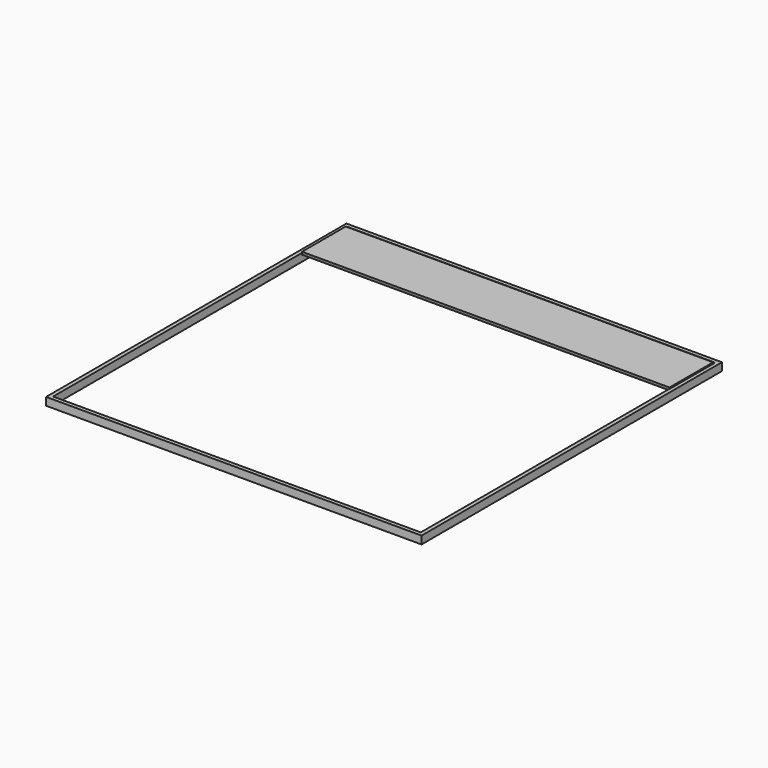
from build123d import *

# Parameters (mm, degrees)
F1_DEPTH  = 19.05
F2_W      = 895.35
F2_H      = 19.05
F5_DEPTH  = 19.05
F6_DEPTH  = 38.1
F3_W      = 895.35
F3_H      = 19.05
F7_DEPTH  = 19.05
F4_W      = 895.35
F4_H      = 19.05
F8_DEPTH  = 127
F10_W     = 895.35
F10_H     = 19.05
F11_DEPTH = 19.05
F12_W     = 895.35
F12_H     = 133.35
F13_DEPTH = 3.175
F13_TAPER = 3


# Not quite as in the source:
# - the program builds the solid bodies; features that only make, move or delete a surface that nothing else refers to are left out


with BuildPart() as f1:
    # F0 (on Top) → F1 (new body)
    with BuildSketch(Plane.XY):
        Polygon((457.2, -457.2), (457.2, 457.2), (186.2517595291, 457.2), (-457.2, 457.2), (-457.2, -457.2), align=None)
        Polygon((-447.675, 447.675), (186.2517595291, 447.675), (447.675, 447.675), (447.675, -447.675), (-447.675, -447.675), align=None, mode=Mode.SUBTRACT)
    extrude(amount=F1_DEPTH)

    # F3 (on face) → F7 (cut)
    with BuildSketch(Plane.XY.offset(19.05)):
        with Locations((0, 298.0556269322)):
            Rectangle(F3_W, F3_H)
    extrude(amount=-F7_DEPTH, mode=Mode.SUBTRACT)

    # F4 (on face) → F8 (cut)
    with BuildSketch(Plane.XY.offset(19.05)):
        with Locations((0, 298.0556269322)):
            Rectangle(F4_W, F4_H)
    extrude(amount=-F8_DEPTH, mode=Mode.SUBTRACT)

    # F10 (on face) → F11 (cut)
    with BuildSketch(Plane.XY.offset(19.05)):
        with Locations((0, 298.0556269322)):
            Rectangle(F10_W, F10_H)
    extrude(amount=-F11_DEPTH, mode=Mode.SUBTRACT)

    # F12 (on face) → F13 (join, symmetric)
    with BuildSketch(Plane.XY.offset(19.05)):
        with Locations((0.6440271378, 375.4221406161)):
            Rectangle(F12_W, F12_H)
    extrude(amount=F13_DEPTH, both=True, taper=F13_TAPER)


with BuildPart() as f5:
    # F2 (on face) → F5 (new body)
    with BuildSketch(Plane.XY.offset(19.05)):
        with Locations((0, 298.0556269322)):
            Rectangle(F2_W, F2_H)
    extrude(amount=F5_DEPTH)

    # F6 (cut): a face of the model
    f6_faces = [f5.faces().sort_by_distance(p)[0] for p in [
        (0, 298.0556269322, 38.1),
    ]]
    extrude(f6_faces, amount=-F6_DEPTH, mode=Mode.SUBTRACT)


solid = f1.part
